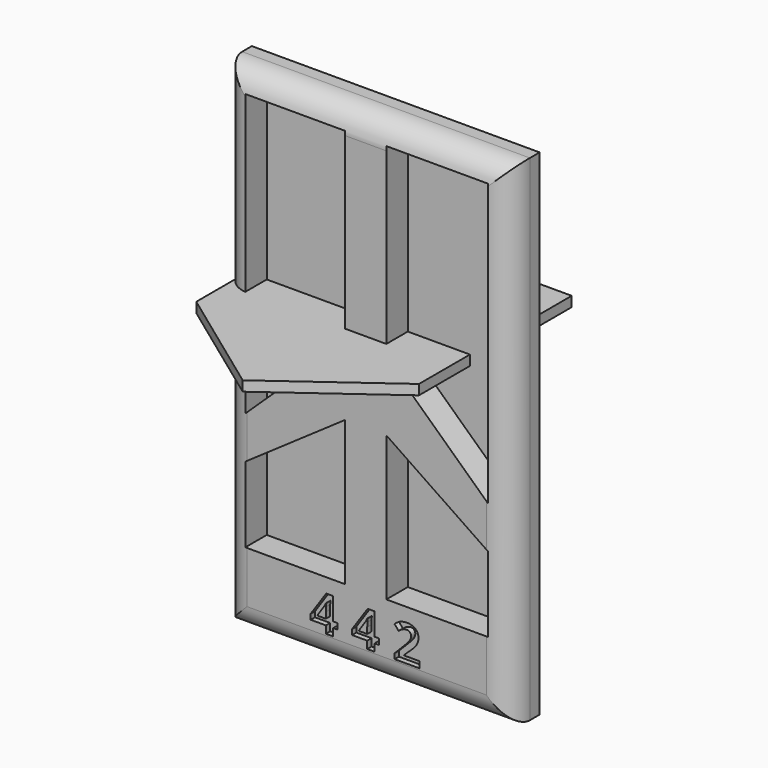
from build123d import *

# Parameters (mm, degrees)
F0_W         = 60.2813165593
F0_H         = 103.6993224955
F1_DEPTH     = 7.62
F2_DEPTH     = 2
F0_W_2       = 50.8
F0_H_2       = 9.3282237438
F3_DEPTH     = 7.62
F0_TEXT_SIZE = 10.4430700756
F4_DEPTH     = 6.5
F5_T1_DEPTH  = 129.0993224955
F5_T3_DEPTH  = 85.6813165593
F6_DEPTH     = 7.62
F7_W         = 46.65
F7_H         = 40
F8_DEPTH     = 2.1


# Not quite as in the source:
# - a fillet or chamfer that OpenCascade refuses, or shapes differently, is made with other operations: its cross-section is extruded or revolved along the edge and cut away or added
# - Text() gives the source's letters only with a copy of the font that has no kerning and outlines rounded to 1/6400 em; it was checked with that copy


with BuildPart() as f1:
    # F0 (on Front) → F1 (new body)
    with BuildSketch(Plane.XZ):
        with Locations((0.0199185564, -9.055939373)):
            Rectangle(F0_W, F0_H)
        Polygon((-25.4000009313, -20.3398931772), (-25.4000009313, 38.5467081877), (-4.5306864195, 38.5467081877), (4.1450969875, 38.5467081877), (25.3999990687, 38.5467081877), (25.3999990687, -20.3398931772), (25.3999990687, -29.2084701359), (25.3999990687, -45.0176782906), (25.3999990687, -47.3750680685), (25.3999990687, -56.7032918123), (-25.4000009313, -56.7032918123), (-25.4000009313, -47.3750680685), (-25.4000009313, -45.0176782906), (-25.4000009313, -29.2084701359), align=None, mode=Mode.SUBTRACT)
        Polygon((4.1450969875, 38.5467081877), (-4.5306864195, 38.5467081877), (-4.5306864195, -0.4819879541), (-25.4000009313, -20.3398931772), (-25.4000009313, -29.2084701359), (-4.5306864195, -14.7488312796), (-4.5306864195, -45.0176782906), (4.1450969875, -45.0176782906), (4.1450969875, -14.7488312796), (25.3999990687, -29.2084701359), (25.3999990687, -20.3398931772), (4.1450969875, -0.4819879541), align=None)
        Polygon((-4.5306864195, -45.0176782906), (-25.4000009313, -45.0176782906), (-25.4000009313, -47.3750680685), (25.3999990687, -47.3750680685), (25.3999990687, -45.0176782906), (4.1450969875, -45.0176782906), align=None)
    extrude(amount=F1_DEPTH)

    # F0 (on Front) → F2 (join)
    with BuildSketch(Plane.XZ):
        Polygon((25.3999990687, 38.5467081877), (4.1450969875, 38.5467081877), (4.1450969875, -0.4819879541), (25.3999990687, -20.3398931772), align=None)
        Polygon((-4.5306864195, 38.5467081877), (-25.4000009313, 38.5467081877), (-25.4000009313, -20.3398931772), (-4.5306864195, -0.4819879541), align=None)
        Polygon((-4.5306864195, -14.7488312796), (-25.4000009313, -29.2084701359), (-25.4000009313, -45.0176782906), (-4.5306864195, -45.0176782906), align=None)
        Polygon((25.3999990687, -45.0176782906), (25.3999990687, -29.2084701359), (4.1450969875, -14.7488312796), (4.1450969875, -45.0176782906), align=None)
    extrude(amount=F2_DEPTH)

    # F0 (on Front) → F3 (join)
    with BuildSketch(Plane.XZ):
        with Locations((-9.313e-07, -52.0391799404)):
            Rectangle(F0_W_2, F0_H_2)
        Polygon((-6.0900417407, -52.6989886995), (-6.0900417407, -53.922785974), (-6.9874930753, -53.922785974), (-6.9874930753, -55.4680339992), (-8.5278459115, -55.4680339992), (-8.5278459115, -53.922785974), (-11.7097188251, -53.922785974), (-11.7097188251, -52.826263616), (-8.4397325077, -48.0126610031), (-6.9874930753, -48.0126610031), (-6.9874930753, -52.6989886995), align=None, mode=Mode.SUBTRACT)
        Polygon((2.5842333408, -52.6989886995), (2.5842333408, -53.922785974), (1.6867820062, -53.922785974), (1.6867820062, -55.4680339992), (0.14642917, -55.4680339992), (0.14642917, -53.922785974), (-3.0354437436, -53.922785974), (-3.0354437436, -52.826263616), (0.2345425738, -48.0126610031), (1.6867820062, -48.0126610031), (1.6867820062, -52.6989886995), align=None, mode=Mode.SUBTRACT)
        with BuildLine():
            Line((11.0904402633, -54.1414377537), (11.0904402633, -55.4680339992))
            Line((11.0904402633, -55.4680339992), (5.8786956037, -55.4680339992))
            Line((5.8786956037, -55.4680339992), (5.8786956037, -54.3715116413))
            Line((5.8786956037, -54.3715116413), (7.7502895688, -52.4803369198))
            add(Edge.make_bspline(
                [(7.7502895688, -52.4803369198), (8.5824717155, -51.6285740167), (8.8370215486, -51.2997804823)],
                knots=[0, 0, 0, 1, 1, 1], degree=2))
            add(Edge.make_bspline(
                [(8.8370215486, -51.2997804823), (9.0915713817, -50.9709869479), (9.2041607309, -50.6903294396)],
                knots=[0, 0, 0, 1, 1, 1], degree=2))
            add(Edge.make_bspline(
                [(9.2041607309, -50.6903294396), (9.3167500802, -50.4096719313), (9.3167500802, -50.1094336667)],
                knots=[0, 0, 0, 1, 1, 1], degree=2))
            add(Edge.make_bspline(
                [(9.3167500802, -50.1094336667), (9.3167500802, -49.6607079994), (9.0687271659, -49.4412403548)],
                knots=[0, 0, 0, 1, 1, 1], degree=2))
            add(Edge.make_bspline(
                [(9.0687271659, -49.4412403548), (8.8207042516, -49.2217727102), (8.4078766376, -49.2217727102)],
                knots=[0, 0, 0, 1, 1, 1], degree=2))
            add(Edge.make_bspline(
                [(8.4078766376, -49.2217727102), (7.9754682673, -49.2217727102), (7.5675358425, -49.4208437336)],
                knots=[0, 0, 0, 1, 1, 1], degree=2))
            add(Edge.make_bspline(
                [(7.5675358425, -49.4208437336), (7.1596034177, -49.6199147569), (6.7157729395, -49.9870539392)],
                knots=[0, 0, 0, 1, 1, 1], degree=2))
            Line((6.7157729395, -49.9870539392), (5.8591148473, -48.9721180663))
            add(Edge.make_bspline(
                [(5.8591148473, -48.9721180663), (6.409007756, -48.5021799129), (6.7712517492, -48.3088199435)],
                knots=[0, 0, 0, 1, 1, 1], degree=2))
            add(Edge.make_bspline(
                [(6.7712517492, -48.3088199435), (7.1334957425, -48.1154599741), (7.5618247886, -48.0110292734)],
                knots=[0, 0, 0, 1, 1, 1], degree=2))
            add(Edge.make_bspline(
                [(7.5618247886, -48.0110292734), (7.9901538346, -47.9065985726), (8.5204659869, -47.9065985726)],
                knots=[0, 0, 0, 1, 1, 1], degree=2))
            add(Edge.make_bspline(
                [(8.5204659869, -47.9065985726), (9.2188462982, -47.9065985726), (9.7540536396, -48.1611484057)],
                knots=[0, 0, 0, 1, 1, 1], degree=2))
            add(Edge.make_bspline(
                [(9.7540536396, -48.1611484057), (10.289260981, -48.4156982388), (10.5854199214, -48.8750301491)],
                knots=[0, 0, 0, 1, 1, 1], degree=2))
            add(Edge.make_bspline(
                [(10.5854199214, -48.8750301491), (10.8815788618, -49.3343620595), (10.8815788618, -49.9250482107)],
                knots=[0, 0, 0, 1, 1, 1], degree=2))
            add(Edge.make_bspline(
                [(10.8815788618, -49.9250482107), (10.8815788618, -50.4406747956), (10.7004568652, -50.8918480575)],
                knots=[0, 0, 0, 1, 1, 1], degree=2))
            add(Edge.make_bspline(
                [(10.7004568652, -50.8918480575), (10.5193348686, -51.3430213194), (10.1391418486, -51.817038797)],
                knots=[0, 0, 0, 1, 1, 1], degree=2))
            add(Edge.make_bspline(
                [(10.1391418486, -51.817038797), (9.7589488287, -52.2910562746), (8.8011234952, -53.1689268529)],
                knots=[0, 0, 0, 1, 1, 1], degree=2))
            Line((8.8011234952, -53.1689268529), (7.841666432, -54.0712733766))
            Line((7.841666432, -54.0712733766), (7.841666432, -54.1414377537))
            Line((7.841666432, -54.1414377537), (11.0904402633, -54.1414377537))
        make_face(mode=Mode.SUBTRACT)
    extrude(amount=F3_DEPTH)

    # F0 (on Front) → F4 (join)
    with BuildSketch(Plane.XZ):
        with Locations((-11.8875773624, -55.4680339992)):
            Text('4 4 2', F0_TEXT_SIZE, font='Open Sans', font_style=FontStyle.BOLD, text_align=(TextAlign.LEFT, TextAlign.BOTTOM))
    extrude(amount=F4_DEPTH)

    # F5: fillet of radius 5.08 on 4 edges, made by hand

    # F5_s2 → F5_t1 (cut)
    with BuildSketch(Plane.XY.offset(-73.6056006207)):
        with BuildLine():
            ThreePointArc((25.080576836, -7.62), (28.6726792845, -6.1321024484), (30.160576836, -2.54))
            Line((30.160576836, -2.54), (30.160576836, -7.62))
            Line((30.160576836, -7.62), (25.080576836, -7.62))
        make_face()
        with BuildLine():
            ThreePointArc((-25.0407397233, -7.62), (-28.6328421717, -6.1321024484), (-30.1207397233, -2.54))
            Line((-30.1207397233, -2.54), (-30.1207397233, -7.62))
            Line((-30.1207397233, -7.62), (-25.0407397233, -7.62))
        make_face()
    extrude(amount=F5_T1_DEPTH, mode=Mode.SUBTRACT)

    # F5_s4 → F5_t3 (cut)
    with BuildSketch(Plane.YZ.offset(-42.8207397233)):
        with BuildLine():
            ThreePointArc((-7.62, -55.8256006207), (-6.1321024484, -59.4177030691), (-2.54, -60.9056006207))
            Line((-2.54, -60.9056006207), (-7.62, -60.9056006207))
            Line((-7.62, -60.9056006207), (-7.62, -55.8256006207))
        make_face()
        with BuildLine():
            ThreePointArc((-7.62, 37.7137218748), (-6.1321024484, 41.3058243232), (-2.54, 42.7937218748))
            Line((-2.54, 42.7937218748), (-7.62, 42.7937218748))
            Line((-7.62, 42.7937218748), (-7.62, 37.7137218748))
        make_face()
    extrude(amount=F5_T3_DEPTH, mode=Mode.SUBTRACT)

    # F0 (on Front) → F6 (join)
    with BuildSketch(Plane.XZ):
        with BuildLine():
            Line((-1.6484734992, -52.6989886995), (0.14642917, -52.6989886995))
            Line((0.14642917, -52.6989886995), (0.14642917, -51.4343981825))
            add(Edge.make_bspline(
                [(0.14642917, -51.4343981825), (0.14642917, -51.1178426208), (0.1725368452, -50.5165502267)],
                knots=[0, 0, 0, 1, 1, 1], degree=2))
            add(Edge.make_bspline(
                [(0.1725368452, -50.5165502267), (0.1986445204, -49.9152578325), (0.2133300877, -49.8173540505)],
                knots=[0, 0, 0, 1, 1, 1], degree=2))
            Line((0.2133300877, -49.8173540505), (0.1725368452, -49.8173540505))
            add(Edge.make_bspline(
                [(0.1725368452, -49.8173540505), (-0.0167437999, -50.2367085832), (-0.2810840112, -50.6332189002)],
                knots=[0, 0, 0, 1, 1, 1], degree=2))
            Line((-0.2810840112, -50.6332189002), (-1.6484734992, -52.6989886995))
        make_face()
        with BuildLine():
            Line((-10.3227485807, -52.6989886995), (-8.5278459115, -52.6989886995))
            Line((-8.5278459115, -52.6989886995), (-8.5278459115, -51.4343981825))
            add(Edge.make_bspline(
                [(-8.5278459115, -51.4343981825), (-8.5278459115, -51.1178426208), (-8.5017382363, -50.5165502267)],
                knots=[0, 0, 0, 1, 1, 1], degree=2))
            add(Edge.make_bspline(
                [(-8.5017382363, -50.5165502267), (-8.4756305611, -49.9152578325), (-8.4609449938, -49.8173540505)],
                knots=[0, 0, 0, 1, 1, 1], degree=2))
            Line((-8.4609449938, -49.8173540505), (-8.5017382363, -49.8173540505))
            add(Edge.make_bspline(
                [(-8.5017382363, -49.8173540505), (-8.6910188814, -50.2367085832), (-8.9553590927, -50.6332189002)],
                knots=[0, 0, 0, 1, 1, 1], degree=2))
            Line((-8.9553590927, -50.6332189002), (-10.3227485807, -52.6989886995))
        make_face()
    extrude(amount=F6_DEPTH)


with BuildPart() as f8:
    # F7 (on Top) → F8 (new body)
    with BuildSketch(Plane.XY):
        with Locations((-6.1570563765, 4.6485891194)):
            Rectangle(F7_W, F7_H)
        Polygon((17.1679436235, -15.3514108806), (-29.4820563765, -15.3514108806), (-6.1570563765, -32.3514108806), align=None)
    extrude(amount=F8_DEPTH)


solid = Compound([f1.part, f8.part])
